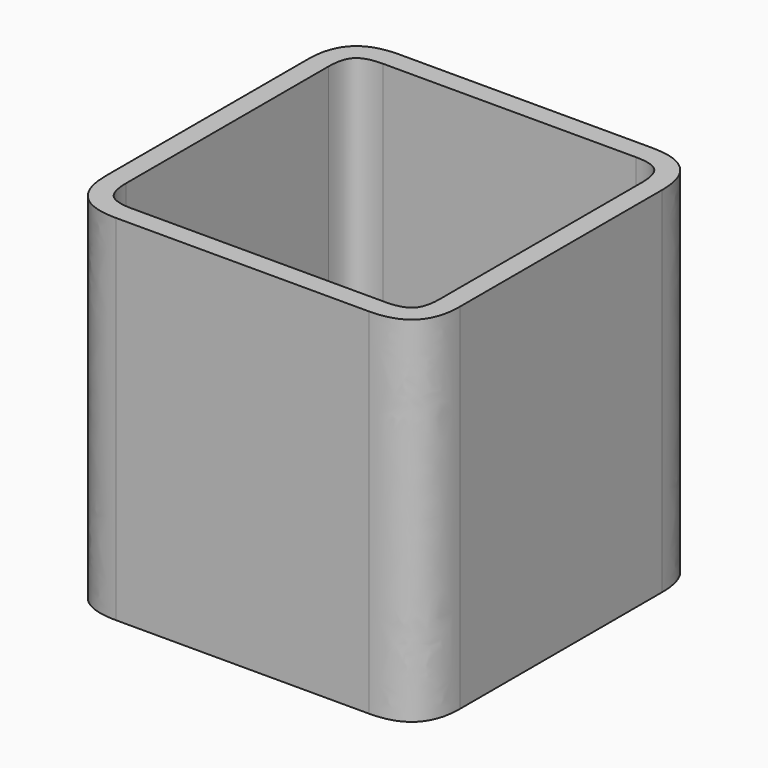
from build123d import *

# Parameters (mm, degrees)
F0_W        = 88.9
F0_H        = 88.9
F1_DEPTH    = 88.9
F2_T1_DEPTH = 152.4
F3_T        = -5.08


# Not quite as in the source:
# - a fillet or chamfer that OpenCascade refuses, or shapes differently, is made with other operations: its cross-section is extruded or revolved along the edge and cut away or added


with BuildPart() as f1:
    # F0 (on Top) → F1 (new body)
    with BuildSketch(Plane.XY):
        Rectangle(F0_W, F0_H)
    extrude(amount=F1_DEPTH)

    # F2: fillet of radius 12.7 on 4 edges, made by hand

    # F2_s2 → F2_t1 (cut)
    with BuildSketch(Plane.XY.offset(-31.75)):
        with BuildLine():
            add(Edge.make_bspline(
                [(31.75, -44.45), (44.45, -44.45), (44.45, -31.75)],
                knots=[0, 0, 0, 1, 1, 1], degree=2, weights=[1, 1, 1]))
            Line((44.45, -31.75), (44.45, -44.45))
            Line((44.45, -44.45), (31.75, -44.45))
        make_face()
        with BuildLine():
            add(Edge.make_bspline(
                [(44.45, 31.75), (44.45, 44.45), (31.75, 44.45)],
                knots=[0, 0, 0, 1, 1, 1], degree=2, weights=[1, 1, 1]))
            Line((31.75, 44.45), (44.45, 44.45))
            Line((44.45, 44.45), (44.45, 31.75))
        make_face()
        with BuildLine():
            add(Edge.make_bspline(
                [(-31.75, -44.45), (-44.45, -44.45), (-44.45, -31.75)],
                knots=[0, 0, 0, 1, 1, 1], degree=2, weights=[1, 1, 1]))
            Line((-44.45, -31.75), (-44.45, -44.45))
            Line((-44.45, -44.45), (-31.75, -44.45))
        make_face()
        with BuildLine():
            add(Edge.make_bspline(
                [(-31.75, 44.45), (-44.45, 44.45), (-44.45, 31.75)],
                knots=[0, 0, 0, 1, 1, 1], degree=2, weights=[1, 1, 1]))
            Line((-44.45, 31.75), (-44.45, 44.45))
            Line((-44.45, 44.45), (-31.75, 44.45))
        make_face()
    extrude(amount=F2_T1_DEPTH, mode=Mode.SUBTRACT)

    # F3
    f3_openings = [f1.faces().sort_by_distance(p)[0] for p in [
        (0, 0, 88.9),
    ]]
    offset(amount=F3_T, openings=f3_openings, kind=Kind.INTERSECTION)


solid = f1.part
